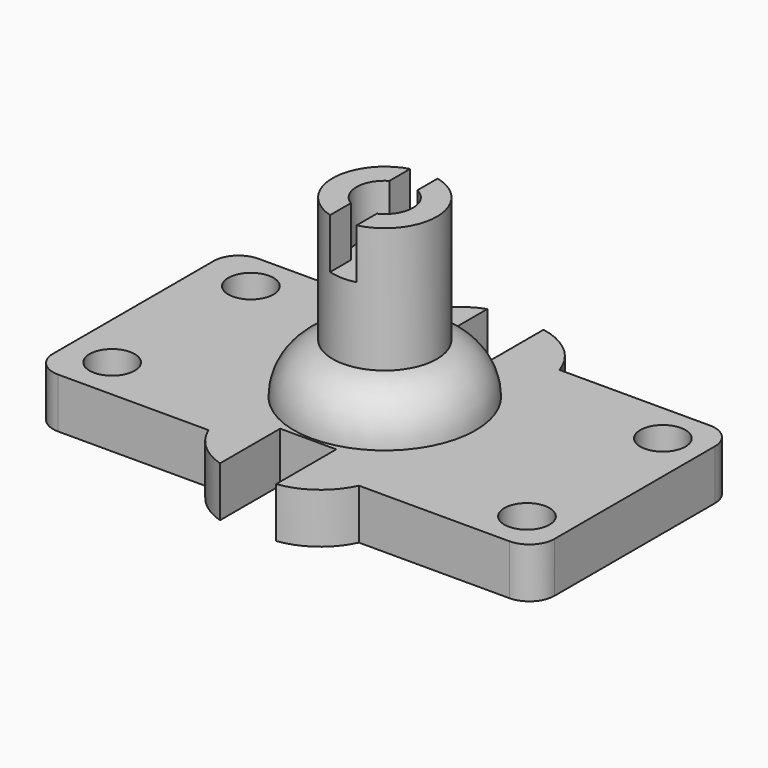
from build123d import *

# Parameters (mm, degrees)
F0_R        = 4.5
F0_W        = 11.19
F0_H        = 12.81
F0_W_2      = 11.1915078014
F0_H_2      = 12.8067285316
F1_DEPTH    = 10
F2_DEPTH    = 15
F3_DEPTH    = 15
F5_DEPTH    = 10
F6_T1_DEPTH = 51.1789036834
F6_T3_DEPTH = 25.0383892744
F6_T6_ANGLE = 359.64
F7_R        = 10.3941452537
F8_DEPTH    = 25
F10_DEPTH   = 10
F11_R       = 5.6272880919
F12_DEPTH   = 10


# Not quite as in the source:
# - a fillet or chamfer that OpenCascade refuses, or shapes differently, is made with other operations: its cross-section is extruded or revolved along the edge and cut away or added


with BuildPart() as f1:
    # F0 (on Top) → F1 (new body)
    with BuildSketch(Plane.XY):
        with BuildLine():
            ThreePointArc((45.4072788358, 26.301991269), (43.9428127417, 29.8375251749), (40.4072788358, 31.301991269))
            Line((40.4072788358, 31.301991269), (10.4072788358, 31.301991269))
            ThreePointArc((10.4072788358, 31.301991269), (6.4487710146, 37.2465605388), (0, 40.315931871))
            Line((0, 40.315931871), (0, 27.505931871))
            Line((0, 27.505931871), (-11.19, 27.505931871))
            Line((-11.19, 27.505931871), (-11.19, 40.315931871))
            ThreePointArc((-11.19, 40.315931871), (-16.4880832553, 36.8313174102), (-19.5927211642, 31.301991269))
            Line((-19.5927211642, 31.301991269), (-49.5927211642, 31.301991269))
            ThreePointArc((-49.5927211642, 31.301991269), (-53.1282550702, 29.8375251749), (-54.5927211642, 26.301991269))
            Line((-54.5927211642, 26.301991269), (-54.5927211642, -13.698008731))
            ThreePointArc((-54.5927211642, -13.698008731), (-53.1282550702, -17.2335426369), (-49.5927211642, -18.698008731))
            Line((-49.5927211642, -18.698008731), (-19.5927211642, -18.698008731))
            ThreePointArc((-19.5927211642, -18.698008731), (-16.2412825657, -23.4529100661), (-11.1915078014, -26.340989396))
            Line((-11.1915078014, -26.340989396), (-11.1915078014, -13.5342608644))
            Line((-11.1915078014, -13.5342608644), (0, -13.5342608644))
            Line((0, -13.5342608644), (0, -26.340989396))
            ThreePointArc((0, -26.340989396), (6.184106324, -23.8545793063), (10.4072788358, -18.698008731))
            Line((10.4072788358, -18.698008731), (40.4072788358, -18.698008731))
            ThreePointArc((40.4072788358, -18.698008731), (43.9428127417, -17.2335426369), (45.4072788358, -13.698008731))
            Line((45.4072788358, -13.698008731), (45.4072788358, 26.301991269))
        make_face()
        with Locations((-45.5849245191, -10.236135684)):
            Circle(F0_R, mode=Mode.SUBTRACT)
        with Locations((37.3101647261, -10.4333672206)):
            Circle(F0_R, mode=Mode.SUBTRACT)
        with Locations((-44.7660312057, 23.3383905143)):
            Circle(F0_R, mode=Mode.SUBTRACT)
        with Locations((37.396017462, 23.3383905143)):
            Circle(F0_R, mode=Mode.SUBTRACT)
        with Locations((-5.595, 33.910931871)):
            Rectangle(F0_W, F0_H)
        with Locations((-5.5957539007, -19.9376251302)):
            Rectangle(F0_W_2, F0_H_2)
    extrude(amount=F1_DEPTH)

    # F2 (cut): a face of the model
    f2_faces = [f1.faces().sort_by_distance(p)[0] for p in [
        (-5.5957539007, -26.340989396, 5),
    ]]
    extrude(f2_faces, amount=-F2_DEPTH, mode=Mode.SUBTRACT)

    # F3 (cut): a face of the model
    f3_faces = [f1.faces().sort_by_distance(p)[0] for p in [
        (-5.595, 40.315931871, 5),
    ]]
    extrude(f3_faces, amount=-F3_DEPTH, mode=Mode.SUBTRACT)

    # F4 (on face) → F5 (join)
    with BuildSketch(Plane.XY.offset(10)):
        with BuildLine():
            Line((-5.186308641, 7.2335354052), (-5.186308641, -10.8872503349))
            ThreePointArc((-5.186308641, -10.8872503349), (7.6270218363, -5.579795072), (12.9344770991, 7.2335354052))
            ThreePointArc((12.9344770991, 7.2335354052), (8.0372600319, 19.6230514326), (-4.0074049576, 25.315931871))
            Line((-4.0074049576, 25.315931871), (-5.186308641, 25.315931871))
            Line((-5.186308641, 25.315931871), (-5.186308641, 7.2335354052))
        make_face()
        with BuildLine():
            ThreePointArc((-6.3652123244, 25.315931871), (-23.2974945196, 6.6437711237), (-5.186308641, -10.8872503349))
            Line((-5.186308641, -10.8872503349), (-5.186308641, 7.2335354052))
            Line((-5.186308641, 7.2335354052), (-5.186308641, 25.315931871))
            Line((-5.186308641, 25.315931871), (-6.3652123244, 25.315931871))
        make_face()
        with BuildLine():
            ThreePointArc((-5.186308641, 25.3543211454), (-5.7760729225, 25.3447212839), (-6.3652123244, 25.315931871))
            Line((-6.3652123244, 25.315931871), (-5.186308641, 25.315931871))
            Line((-5.186308641, 25.315931871), (-5.186308641, 25.3543211454))
        make_face()
    extrude(amount=F5_DEPTH)

    # F6: fillet of radius 10 on 3 edges, made by hand

    # F6_s2 → F6_t1 (cut)
    with BuildSketch(Plane.YZ.offset(-30.186308641)):
        with BuildLine():
            ThreePointArc((25.315931871, 10), (22.3869996828, 17.0710678119), (15.315931871, 20))
            Line((15.315931871, 20), (15.315931871, 20.2))
            Line((15.315931871, 20.2), (25.515931871, 20.2))
            Line((25.515931871, 20.2), (25.515931871, 10))
            Line((25.515931871, 10), (25.315931871, 10))
        make_face()
    extrude(amount=F6_T1_DEPTH, mode=Mode.SUBTRACT)

    # F6_s4 → F6_t3 (cut)
    with BuildSketch(Plane.XZ.offset(-50.3543211454)):
        with BuildLine():
            ThreePointArc((-5.186308641, 10), (-8.1152408291, 17.0710678119), (-15.186308641, 20))
            Line((-15.186308641, 20), (-15.186308641, 20.2))
            Line((-15.186308641, 20.2), (-4.986308641, 20.2))
            Line((-4.986308641, 20.2), (-4.986308641, 10))
            Line((-4.986308641, 10), (-5.186308641, 10))
        make_face()
    extrude(amount=F6_T3_DEPTH, mode=Mode.SUBTRACT)

    # F6_s5 → F6_t6 (revolve, cut)
    with BuildSketch(Plane(origin=(-5.394442731, 0.1586987059, 0), x_dir=(0, 0, 1), z_dir=(0.9995675441, -0.0294062026, 0))):
        with BuildLine():
            ThreePointArc((10, -25.1986833179), (17.0710678119, -22.2697511298), (20, -15.1986833179))
            Line((20, -15.1986833179), (20.2, -15.1986833179))
            Line((20.2, -15.1986833179), (20.2, -25.3986833179))
            Line((20.2, -25.3986833179), (10, -25.3986833179))
            Line((10, -25.3986833179), (10, -25.1986833179))
        make_face()
    revolve(axis=Axis((-5.186308641, 7.2335354052, 20), (0, 0, 1)), revolution_arc=F6_T6_ANGLE, mode=Mode.SUBTRACT)

    # F7 (on face) → F8 (join)
    with BuildSketch(Plane.XY.offset(20)):
        with Locations((-5.186308641, 7.2335354052)):
            Circle(F7_R)
    extrude(amount=F8_DEPTH)

    # F9 (on face) → F10 (cut)
    with BuildSketch(Plane.XY.offset(45)):
        with BuildLine():
            Line((-2.7313069579, -2.866525104), (-2.7313069579, 17.3335959145))
            ThreePointArc((-2.7313069579, 17.3335959145), (-5.4257935051, 17.6249213838), (-8.1039983469, 17.2097742925))
            Line((-8.1039983469, 17.2097742925), (-8.1039983469, -2.742703482))
            ThreePointArc((-8.1039983469, -2.742703482), (-5.4257935051, -3.1578505733), (-2.7313069579, -2.866525104))
        make_face()
    extrude(amount=-F10_DEPTH, mode=Mode.SUBTRACT)

    # F11 (on face) → F12 (cut)
    with BuildSketch(Plane.XY.offset(45)):
        with Locations((-5.186308641, 7.2335354052)):
            Circle(F11_R)
    extrude(amount=-F12_DEPTH, mode=Mode.SUBTRACT)


solid = f1.part
